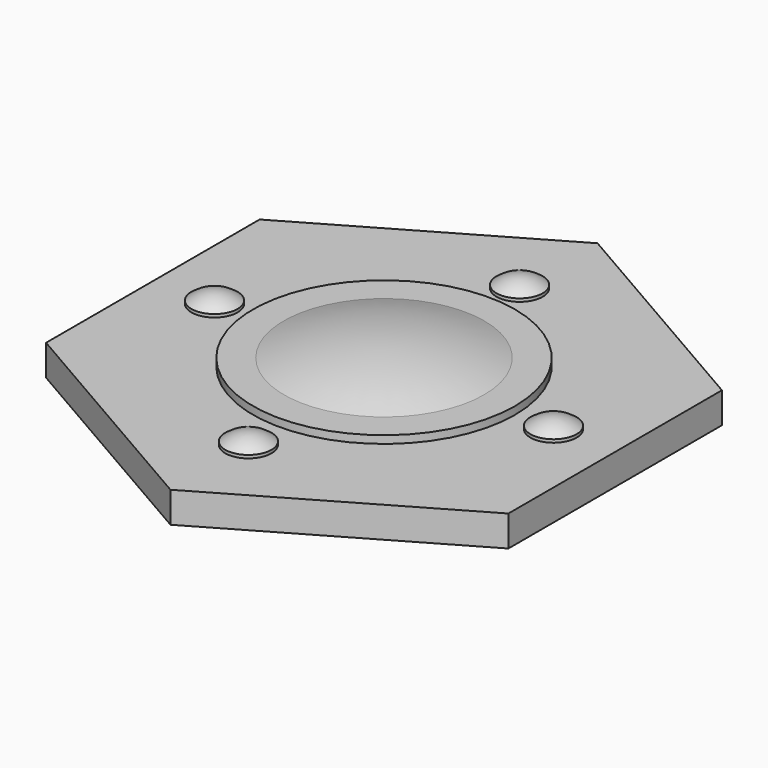
from build123d import *

# Parameters (mm, degrees)
F0_R     = 0.75
F0_R_2   = 7.5
F1_DEPTH = 2
F6_COUNT = 4


with BuildPart() as f1:
    # F0 (on Top) → F1 (new body)
    with BuildSketch(Plane.XY):
        Polygon((15, -8.6602540378), (15, 8.6602540378), (0, 17.3205080757), (-15, 8.6602540378), (-15, -8.6602540378), (0, -17.3205080757), align=None)
        with Locations((0, -11)):
            Circle(F0_R, mode=Mode.SUBTRACT)
        with Locations((-11, 0)):
            Circle(F0_R, mode=Mode.SUBTRACT)
        Circle(F0_R_2, mode=Mode.SUBTRACT)
        with Locations((11, 0)):
            Circle(F0_R, mode=Mode.SUBTRACT)
        with Locations((0, 11)):
            Circle(F0_R, mode=Mode.SUBTRACT)
    extrude(amount=F1_DEPTH)


with BuildPart() as f3:
    # F2 (on Front) → F3 (revolve)
    with BuildSketch(Plane.XZ):
        with BuildLine():
            Line((8.5, 2), (8.5, 2.5))
            Line((8.5, 2.5), (6.5, 2.5))
            ThreePointArc((6.5, 2.5), (3.3010833884, 3.365480662), (0, 3.6569814812))
            Line((0, 3.6569814812), (0, -2))
            Line((0, -2), (8.5, -2))
            Line((8.5, -2), (8.5, -1))
            Line((8.5, -1), (10, 0))
            Line((10, 0), (7.5, 0))
            Line((7.5, 0), (7.5, 2))
            Line((7.5, 2), (8.5, 2))
        make_face()
    revolve(axis=Axis((0, 0, 0.8284907406), (0, 0, -1)))


with BuildPart() as f5:
    # F4 (on Front) → F5 (revolve)
    with BuildSketch(Plane.XZ):
        with BuildLine():
            Line((12.5, 2), (12.5, 2.2))
            ThreePointArc((12.5, 2.2), (11.7957485211, 2.5949511868), (11, 2.7318485081))
            Line((11, 2.7318485081), (11, -2.2681514919))
            Line((11, -2.2681514919), (11.75, -2.2681514919))
            Line((11.75, -2.2681514919), (11.75, 2))
            Line((11.75, 2), (12.5, 2))
        make_face()
    revolve(axis=Axis((11, 0, 0.2318485081), (0, 0, 1)))


with BuildPart() as f6_1:
    # F6: instance of F5
    add(f5.part.rotate(Axis((0, 0, 0.8730492555), (0, 0, -1)), 1 * 360 / F6_COUNT))


with BuildPart() as f6_2:
    # F6: instance of F5
    add(f5.part.rotate(Axis((0, 0, 0.8730492555), (0, 0, -1)), 2 * 360 / F6_COUNT))


with BuildPart() as f6_3:
    # F6: instance of F5
    add(f5.part.rotate(Axis((0, 0, 0.8730492555), (0, 0, -1)), 3 * 360 / F6_COUNT))


solid = Compound([f1.part, f3.part, f5.part, f6_1.part, f6_2.part, f6_3.part])
